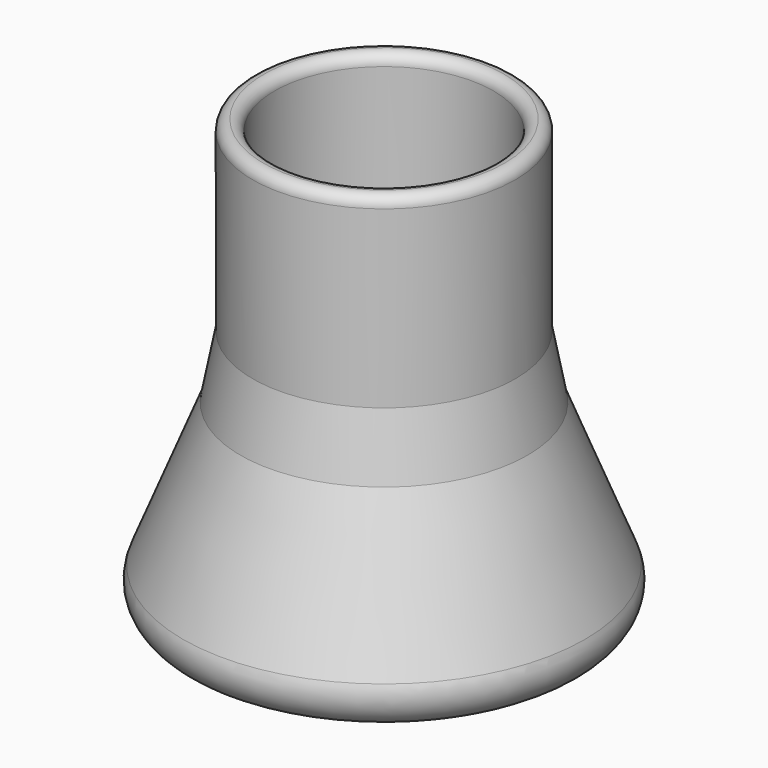
from build123d import *

# Parameters (mm, degrees)
F0_R     = 50
F2_R     = 30
F4_DEPTH = 50
F5_T     = -5
F6_R     = 2.49999
F7_R     = 7.5
F8_SIZE  = 7.5


# Not quite as in the source:
# - a fillet or chamfer is up to 0.001 mm smaller than in the source, because OpenCascade refuses the exact size


with BuildPart() as f3:
    # F0 (on Top) → F3 section 0
    with BuildSketch(Plane.XY):
        Circle(F0_R)
    # F2 (on offset) → F3 section 1
    with BuildSketch(Plane.XY.offset(50)):
        Circle(F2_R)
    loft()

    # F4 (add): a face of the model
    f4_faces = [f3.faces().sort_by_distance(p)[0] for p in [
        (0, 0, 50),
    ]]
    extrude(f4_faces, amount=F4_DEPTH)

    # F5
    f5_openings = [f3.faces().sort_by_distance(p)[0] for p in [
        (0, 0, 100),
    ]]
    offset(amount=F5_T, openings=f5_openings, kind=Kind.INTERSECTION)

    # F6 (radius 2.5 in the source; OpenCascade refuses exactly that, so slightly less here)
    f6_edges = [f3.edges().sort_by_distance(p)[0] for p in [
        (-30, 0, 100),
        (-25, 0, 100),
    ]]
    fillet(f6_edges, radius=F6_R)

    # F7
    f7_edges = [f3.edges().sort_by_distance(p)[0] for p in [
        (-50, 0, 0),
        (-42.614835, 0, 5),
    ]]
    fillet(f7_edges, radius=F7_R)

    # F8
    f8_edges = [f3.edges().sort_by_distance(p)[0] for p in [
        (-30, 0, 50),
        (-25, 0, 49.037088),
    ]]
    chamfer(f8_edges, length=F8_SIZE)


solid = f3.part
